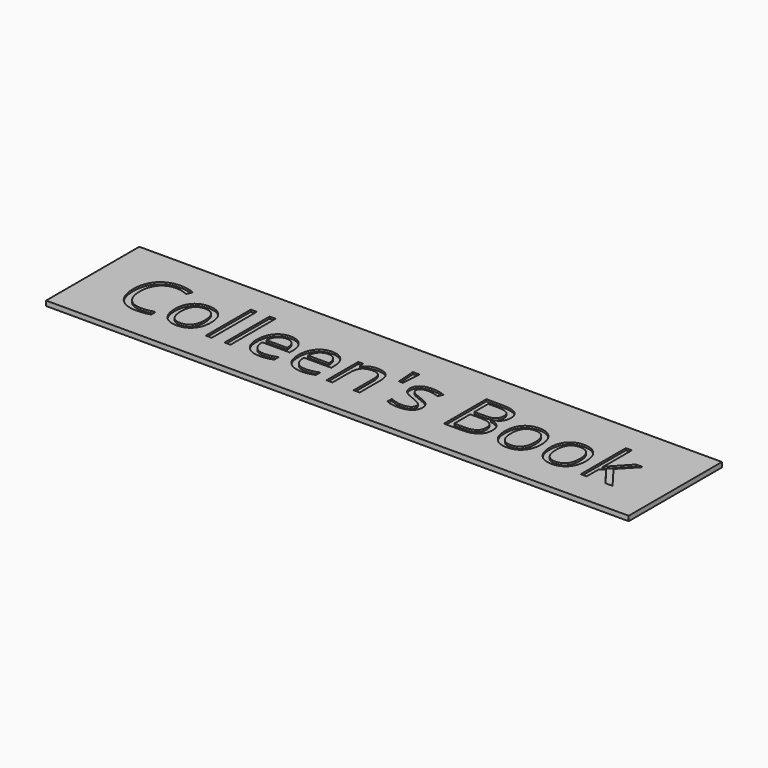
from build123d import *

# Parameters (mm, degrees)
F0_W         = 120
F0_H         = 24
F1_DEPTH     = 1
F2_TEXT_SIZE = 15.2777777778
F3_DEPTH     = 0.4


# Not quite as in the source:
# - Text() gives the source's letters only with a copy of the font that has no kerning and outlines rounded to 1/6400 em; it was checked with that copy


with BuildPart() as f1:
    # F0 (on Top) → F1 (new body)
    with BuildSketch(Plane.XY):
        Rectangle(F0_W, F0_H)
    extrude(amount=F1_DEPTH)

    # F2 (on face) → F3 (cut)
    with BuildSketch(Plane.XY.offset(1)):
        with Locations((-52.5, -5.5)):
            Text("Colleen's Book", F2_TEXT_SIZE, font='Open Sans', text_align=(TextAlign.LEFT, TextAlign.BOTTOM))
    extrude(amount=-F3_DEPTH, mode=Mode.SUBTRACT)


solid = f1.part
